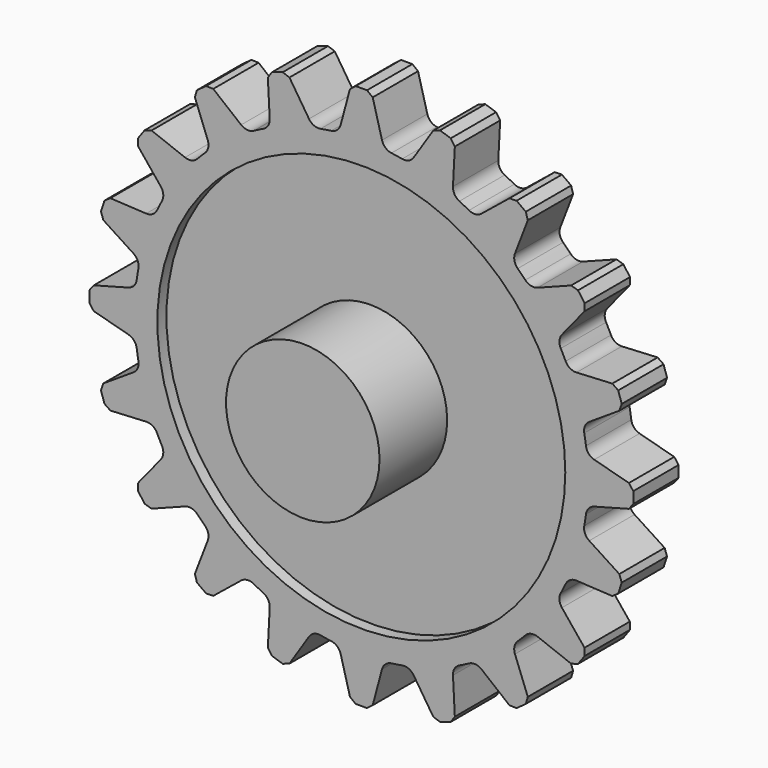
from build123d import *

# Parameters (mm, degrees)
F0_R            = 100
F1_DEPTH        = 25
F3_DEPTH        = 25
F3_COPIES_COUNT = 20
F4_SIZE         = 2
F5_R            = 5
F6_R            = 90
F7_DEPTH        = 5
F8_DEPTH        = 5
F9_DEPTH        = 5
F10_DEPTH       = 10
F11_R           = 33.8638669845
F12_DEPTH       = 37.3


# Not quite as in the source:
# - a pattern or mirror of a feature is missing from the dataset's text; its kind, count and spacing are read off the source's solid


with BuildPart() as f1:
    # F0 (on Front) → F1 (new body)
    with BuildSketch(Plane.XZ):
        Circle(F0_R)
    extrude(amount=F1_DEPTH)

    # F2 (on Front) → F3 (join)
    with BuildSketch(Plane.XZ):
        Polygon((-4.5, 120), (-9.9931095726, 99.4994359837), (9.9931095726, 99.4994359837), (4.5, 120), align=None)
    f3 = extrude(amount=F3_DEPTH)

    # F3_copies: F3 ×20 about axis
    f3_copies_axis = Axis((0, 0, 0), (0, 1, 0))
    for i in range(1, F3_COPIES_COUNT):
        add(f3.rotate(f3_copies_axis, i * 360 / F3_COPIES_COUNT))

    # F4
    f4_edges = [f1.edges().sort_by_distance(p)[0] for p in [
        (4.5, -12.5, 120),
        (-4.5, -12.5, 120),
        (-32.802285, -12.5, 115.517358),
        (115.517358, -12.5, 32.802285),
        (120, -12.5, 4.5),
        (120, -12.5, -4.5),
        (115.517358, -12.5, -32.802285),
        (112.736205, -12.5, -41.361794),
        (99.727073, -12.5, -66.893654),
        (94.437006, -12.5, -74.174807),
        (74.174807, -12.5, -94.437006),
        (66.893654, -12.5, -99.727073),
        (41.361794, -12.5, -112.736205),
        (32.802285, -12.5, -115.517358),
        (4.5, -12.5, -120),
        (-4.5, -12.5, -120),
        (-32.802285, -12.5, -115.517358),
        (-41.361794, -12.5, -112.736205),
        (-66.893654, -12.5, -99.727073),
        (-74.174807, -12.5, -94.437006),
        (-94.437006, -12.5, -74.174807),
        (-99.727073, -12.5, -66.893654),
        (-112.736205, -12.5, -41.361794),
        (-115.517358, -12.5, -32.802285),
        (-120, -12.5, -4.5),
        (-120, -12.5, 4.5),
        (-115.517358, -12.5, 32.802285),
        (-112.736205, -12.5, 41.361794),
        (-99.727073, -12.5, 66.893654),
        (-94.437006, -12.5, 74.174807),
        (-74.174807, -12.5, 94.437006),
        (-66.893654, -12.5, 99.727073),
        (32.802285, -12.5, 115.517358),
        (41.361794, -12.5, 112.736205),
        (66.893654, -12.5, 99.727073),
        (74.174807, -12.5, 94.437006),
        (94.437006, -12.5, 74.174807),
        (99.727073, -12.5, 66.893654),
        (112.736205, -12.5, 41.361794),
        (-41.361794, -12.5, 112.736205),
    ]]
    chamfer(f4_edges, length=F4_SIZE)

    # F5
    f5_edges = [f1.edges().sort_by_distance(p)[0] for p in [
        (-9.99311, -12.5, 99.499436),
        (9.99311, -12.5, 99.499436),
        (97.717628, -12.5, 21.243005),
        (99.499436, -12.5, 9.99311),
        (91.541546, -12.5, 40.251029),
        (86.370537, -12.5, 50.399706),
        (99.499436, -12.5, -9.99311),
        (97.717628, -12.5, -21.243005),
        (74.622932, -12.5, 66.568897),
        (66.568897, -12.5, 74.622932),
        (91.541546, -12.5, -40.251029),
        (86.370537, -12.5, -50.399706),
        (50.399706, -12.5, 86.370537),
        (40.251029, -12.5, 91.541546),
        (74.622932, -12.5, -66.568897),
        (66.568897, -12.5, -74.622932),
        (21.243005, -12.5, 97.717628),
        (50.399706, -12.5, -86.370537),
        (40.251029, -12.5, -91.541546),
        (-21.243005, -12.5, 97.717628),
        (21.243005, -12.5, -97.717628),
        (9.99311, -12.5, -99.499436),
        (-40.251029, -12.5, 91.541546),
        (-50.399706, -12.5, 86.370537),
        (-9.99311, -12.5, -99.499436),
        (-21.243005, -12.5, -97.717628),
        (-66.568897, -12.5, 74.622932),
        (-74.622932, -12.5, 66.568897),
        (-40.251029, -12.5, -91.541546),
        (-50.399706, -12.5, -86.370537),
        (-86.370537, -12.5, 50.399706),
        (-91.541546, -12.5, 40.251029),
        (-66.568897, -12.5, -74.622932),
        (-74.622932, -12.5, -66.568897),
        (-97.717628, -12.5, 21.243005),
        (-99.499436, -12.5, 9.99311),
        (-86.370537, -12.5, -50.399706),
        (-91.541546, -12.5, -40.251029),
        (-99.499436, -12.5, -9.99311),
        (-97.717628, -12.5, -21.243005),
    ]]
    fillet(f5_edges, radius=F5_R)

    # F6 (on face) → F7 (join)
    with BuildSketch(Plane.XZ.offset(25)):
        Circle(F6_R)
    extrude(amount=F7_DEPTH)

    # F8 (add): a face of the model
    f8_faces = [f1.faces().sort_by_distance(p)[0] for p in [
        (0, -30, 0),
    ]]
    extrude(f8_faces, amount=F8_DEPTH)

    # F9 (cut): a face of the model
    f9_faces = [f1.faces().sort_by_distance(p)[0] for p in [
        (0, -35, 0),
    ]]
    extrude(f9_faces, amount=-F9_DEPTH, mode=Mode.SUBTRACT)

    # F10 (cut): a face of the model
    f10_faces = [f1.faces().sort_by_distance(p)[0] for p in [
        (0, -30, 0),
    ]]
    extrude(f10_faces, amount=-F10_DEPTH, mode=Mode.SUBTRACT)

    # F11 (on face) → F12 (join)
    with BuildSketch(Plane.XZ.offset(20)):
        Circle(F11_R)
    extrude(amount=F12_DEPTH)


solid = f1.part
